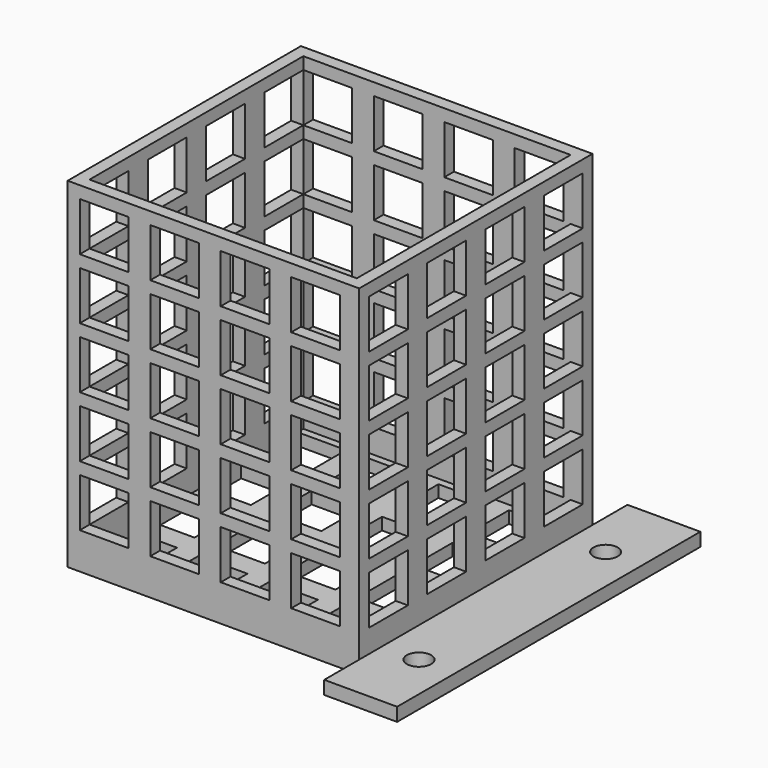
from build123d import *

# Parameters (mm, degrees)
F0_W        = 15
F0_H        = 2.75
F1_DEPTH    = 39
F2_R        = 2.5
F3_DEPTH    = 2.751
F4_W        = 60
F4_H        = 60
F5_DEPTH    = 70
F6_T        = 2.5
F6_T3_DEPTH = 65
F6_T5_DEPTH = 7.75
F7_W        = 10
F7_H        = 10
F8_DEPTH    = 60.001
F9_W        = 10
F9_H        = 10
F10_DEPTH   = 69.001
F11_W       = 10
F11_H       = 10
F12_DEPTH   = 70.001


# Not quite as in the source:
# - a shell that OpenCascade refuses in one call is made with other operations: the cavity is built on its own and cut out
# - a feature names something its author has since deleted; it is built from what else it names


with BuildPart() as f1:
    # F0 (on Front) → F1 (new body, symmetric)
    with BuildSketch(Plane.XZ):
        with Locations((40.5240737289, 19.7500738595)):
            Rectangle(F0_W, F0_H)
    extrude(amount=F1_DEPTH, both=True)

    # F2 (on face) → F3 (cut, through all)
    with BuildSketch(Plane.XY.offset(21.1250738595)):
        with Locations((40.5240737289, 24)):
            Circle(F2_R)
        with Locations((40.5240737289, -24)):
            Circle(F2_R)
    extrude(amount=-F3_DEPTH, mode=Mode.SUBTRACT)

    # F4 (on face) → F5 (join)
    with BuildSketch(Plane(origin=(0, 0, 18.3750738595), x_dir=(1, 0, 0), z_dir=(0, 0, -1))):
        with Locations((3.0240737289, 0)):
            Rectangle(F4_W, F4_H)
    extrude(amount=-F5_DEPTH)

    # F6: shell of thickness 2.5, made by hand


with BuildPart() as f6_core1:
    # F6_t2: copy of F1
    add(f1.part)

    # the walls: a layer under each face that stays
    f6_faces = [f6_core1.faces().sort_by_distance(p)[0] for p in [
        (40.5240737289, 0, 21.1250738595),
        (40.5240737289, 39, 19.7500738595),
        (48.0240737289, 0, 19.7500738595),
        (33.0240737289, 34.5, 19.7500738595),
        (33.0240737289, 0, 54.7500738595),
        (33.0240737289, -34.5, 19.7500738595),
        (40.5240737289, -39, 19.7500738595),
        (38.0240737289, 24, 19.7500738595),
        (38.0240737289, -24, 19.7500738595),
        (10.5240737289, 0, 18.3750738595),
        (3.0240737289, 30, 53.3750738595),
        (3.0240737289, -30, 53.3750738595),
        (-26.9759262711, 0, 53.3750738595),
    ]]
    thicken(f6_faces, amount=-F6_T, mode=Mode.SUBTRACT)

    # F6_s4 → F6_t3 (cut)
    with BuildSketch(Plane.XZ.offset(-32.5)):
        Polygon((33.0490737289, 21.1500738595), (33.0240737289, 18.6250738595), (30.5240737289, 18.6250738595), (30.5240737289, 21.1250738595), align=None)
    extrude(amount=F6_T3_DEPTH, mode=Mode.SUBTRACT)

    # F6_s6 → F6_t5 (cut)
    with BuildSketch(Plane.XY.offset(15.8750738595)):
        Polygon((32.9990737289, 30.025), (35.5240737289, 30), (35.5240737289, 27.5), (33.0240737289, 27.5), align=None)
        Polygon((32.9990737289, -30.025), (35.5240737289, -30), (35.5240737289, -27.5), (33.0240737289, -27.5), align=None)
    extrude(amount=F6_T5_DEPTH, mode=Mode.SUBTRACT)


with BuildPart() as f1_1:
    add(f1.part)

    # what is left inside the walls is the cavity
    f6_cavity = [f6_core1.part.solids().sort_by_distance(p)[0] for p in [
        (3.024074, -27.475, 65.875074),
    ]]
    add(f6_cavity, mode=Mode.SUBTRACT)

    # F7 (on face) → F8 (cut, through all)
    with BuildSketch(Plane.YZ.offset(33.0240737289)):
        with Locations((-22.5, 80.8750738595)):
            Rectangle(F7_W, F7_H)
        with Locations((-7.5, 80.8750738595)):
            Rectangle(F7_W, F7_H)
        with Locations((7.5, 80.8750738595)):
            Rectangle(F7_W, F7_H)
        with Locations((22.5, 80.8750738595)):
            Rectangle(F7_W, F7_H)
        with Locations((22.5, 68.3750738595)):
            Rectangle(F7_W, F7_H)
        with Locations((-22.5, 68.3750738595)):
            Rectangle(F7_W, F7_H)
        with Locations((-7.5, 68.3750738595)):
            Rectangle(F7_W, F7_H)
        with Locations((7.5, 68.3750738595)):
            Rectangle(F7_W, F7_H)
        with Locations((7.5, 55.8750738595)):
            Rectangle(F7_W, F7_H)
        with Locations((22.5, 55.8750738595)):
            Rectangle(F7_W, F7_H)
        with Locations((-7.5, 55.8750738595)):
            Rectangle(F7_W, F7_H)
        with Locations((-22.5, 55.8750738595)):
            Rectangle(F7_W, F7_H)
        with Locations((-22.5, 43.3750738595)):
            Rectangle(F7_W, F7_H)
        with Locations((-7.5, 43.3750738595)):
            Rectangle(F7_W, F7_H)
        with Locations((-7.5, 30.8750738595)):
            Rectangle(F7_W, F7_H)
        with Locations((-22.5, 30.8750738595)):
            Rectangle(F7_W, F7_H)
        with Locations((7.5, 43.3750738595)):
            Rectangle(F7_W, F7_H)
        with Locations((7.5, 30.8750738595)):
            Rectangle(F7_W, F7_H)
        with Locations((22.5, 30.8750738595)):
            Rectangle(F7_W, F7_H)
        with Locations((22.5, 43.3750738595)):
            Rectangle(F7_W, F7_H)
    extrude(amount=-F8_DEPTH, mode=Mode.SUBTRACT)

    # F9 (on face) → F10 (cut, through all)
    with BuildSketch(Plane.XZ.offset(30)):
        with Locations((-19.4759262711, 80.8750738595)):
            Rectangle(F9_W, F9_H)
        with Locations((-4.9759262711, 80.8750738595)):
            Rectangle(F9_W, F9_H)
        with Locations((-4.9759262711, 68.3750738595)):
            Rectangle(F9_W, F9_H)
        with Locations((-19.4759262711, 68.3750738595)):
            Rectangle(F9_W, F9_H)
        with Locations((-4.9759262711, 55.8750738595)):
            Rectangle(F9_W, F9_H)
        with Locations((-19.4759262711, 55.8750738595)):
            Rectangle(F9_W, F9_H)
        with Locations((-19.4759262711, 43.3750738595)):
            Rectangle(F9_W, F9_H)
        with Locations((-4.9759262711, 43.3750738595)):
            Rectangle(F9_W, F9_H)
        with Locations((-4.9759262711, 30.8750738595)):
            Rectangle(F9_W, F9_H)
        with Locations((-19.4759262711, 30.8750738595)):
            Rectangle(F9_W, F9_H)
        with Locations((9.5240737289, 80.8750738595)):
            Rectangle(F9_W, F9_H)
        with Locations((24.0240737289, 80.8750738595)):
            Rectangle(F9_W, F9_H)
        with Locations((24.0240737289, 68.3750738595)):
            Rectangle(F9_W, F9_H)
        with Locations((9.5240737289, 68.3750738595)):
            Rectangle(F9_W, F9_H)
        with Locations((9.5240737289, 55.8750738595)):
            Rectangle(F9_W, F9_H)
        with Locations((24.0240737289, 55.8750738595)):
            Rectangle(F9_W, F9_H)
        with Locations((9.5240737289, 43.3750738595)):
            Rectangle(F9_W, F9_H)
        with Locations((24.0240737289, 43.3750738595)):
            Rectangle(F9_W, F9_H)
        with Locations((24.0240737289, 30.8750738595)):
            Rectangle(F9_W, F9_H)
        with Locations((9.5240737289, 30.8750738595)):
            Rectangle(F9_W, F9_H)
    extrude(amount=-F10_DEPTH, mode=Mode.SUBTRACT)

    # F11 (on face) → F12 (cut, through all)
    with BuildSketch(Plane(origin=(0, 0, 18.3750738595), x_dir=(1, 0, 0), z_dir=(0, 0, -1))):
        with Locations((-19.4759262711, 22.5)):
            Rectangle(F11_W, F11_H)
        with Locations((-19.4759262711, 8)):
            Rectangle(F11_W, F11_H)
        with Locations((-19.4759262711, -6.5)):
            Rectangle(F11_W, F11_H)
        with Locations((-19.4759262711, -21)):
            Rectangle(F11_W, F11_H)
        with Locations((-4.9759262711, 22.5)):
            Rectangle(F11_W, F11_H)
        with Locations((-4.9759262711, 8)):
            Rectangle(F11_W, F11_H)
        with Locations((-4.9759262711, -6.5)):
            Rectangle(F11_W, F11_H)
        with Locations((-4.9759262711, -21)):
            Rectangle(F11_W, F11_H)
        with Locations((9.5240737289, 22.5)):
            Rectangle(F11_W, F11_H)
        with Locations((9.5240737289, 8)):
            Rectangle(F11_W, F11_H)
        with Locations((9.5240737289, -6.5)):
            Rectangle(F11_W, F11_H)
        with Locations((9.5240737289, -21)):
            Rectangle(F11_W, F11_H)
        with Locations((24.0240737289, 22.5)):
            Rectangle(F11_W, F11_H)
        with Locations((24.0240737289, 8)):
            Rectangle(F11_W, F11_H)
        with Locations((24.0240737289, -6.5)):
            Rectangle(F11_W, F11_H)
        with Locations((24.0240737289, -21)):
            Rectangle(F11_W, F11_H)
    extrude(amount=-F12_DEPTH, mode=Mode.SUBTRACT)


solid = f1_1.part
